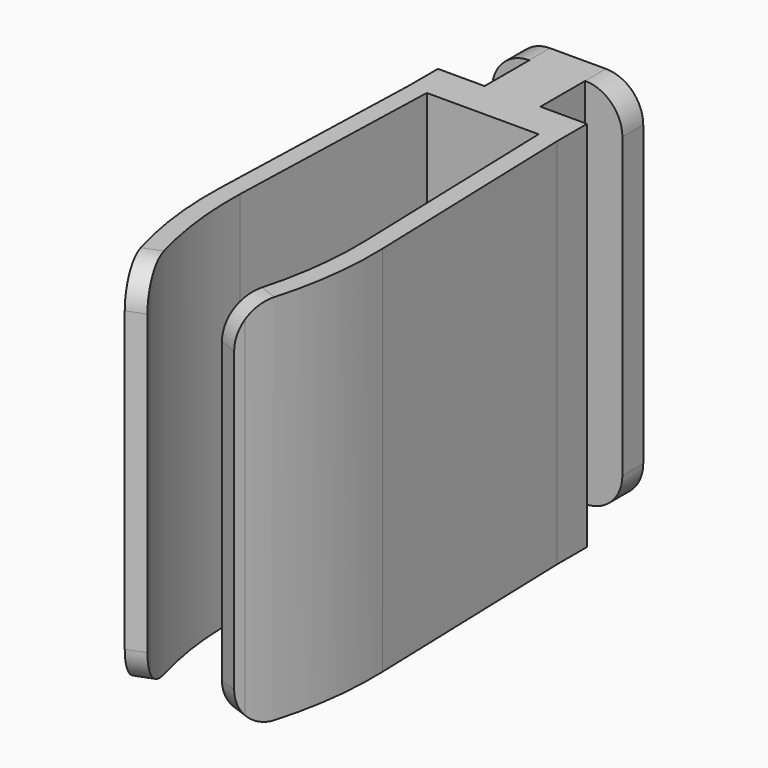
from build123d import *

# Parameters (mm, degrees)
F0_W     = 7
F0_H     = 20
F1_DEPTH = 1.4
F2_W     = 3
F2_H     = 20
F3_DEPTH = 3
F4_W     = 8
F4_H     = 20
F5_DEPTH = 2
F8_DEPTH = 20
F9_R     = 20
F10_R    = 2


# Not quite as in the source:
# - a feature of the source that left no trace in its solid (it failed there, or was rolled back) is left out


with BuildPart() as f1:
    # F0 (on Front) → F1 (new body)
    with BuildSketch(Plane.XZ):
        Rectangle(F0_W, F0_H)
    extrude(amount=F1_DEPTH)

    # F2 (on face) → F3 (join)
    with BuildSketch(Plane.XZ.offset(1.4)):
        Rectangle(F2_W, F2_H)
    extrude(amount=F3_DEPTH)

    # F4 (on face) → F5 (join)
    with BuildSketch(Plane.XZ.offset(4.4)):
        Rectangle(F4_W, F4_H)
    extrude(amount=F5_DEPTH)

    # F7 (on face) → F8 (join, through all)
    with BuildSketch(Plane.XY.offset(10)):
        Polygon((-2.9995108826, -6.4), (-4, -6.4), (-4.5057272064, -22.5674550383), (-2.9367871525, -26.7512951822), (-2, -26.4), (-3.5, -22.4), align=None)
        Polygon((4, -6.4), (2.9995108826, -6.4), (3.5, -22.4), (2, -26.4), (2.9367871525, -26.7512951822), (4.5057272064, -22.5674550383), align=None)
    extrude(amount=-F8_DEPTH)

    # F9
    f9_edges = [f1.edges().sort_by_distance(p)[0] for p in [
        (-3.5, -22.4, 0),
        (3.5, -22.4, 0),
        (4.505727, -22.567455, 0),
        (-4.505727, -22.567455, 0),
    ]]
    fillet(f9_edges, radius=F9_R)

    # F10
    f10_edges = [f1.edges().sort_by_distance(p)[0] for p in [
        (-2.468394, -26.575648, 10),
        (2.468394, -26.575648, 10),
        (-2.468394, -26.575648, -10),
        (2.468394, -26.575648, -10),
        (-3.5, -0.7, -10),
        (3.5, -0.7, -10),
        (-3.5, -0.7, 10),
        (3.5, -0.7, 10),
    ]]
    fillet(f10_edges, radius=F10_R)


solid = f1.part
